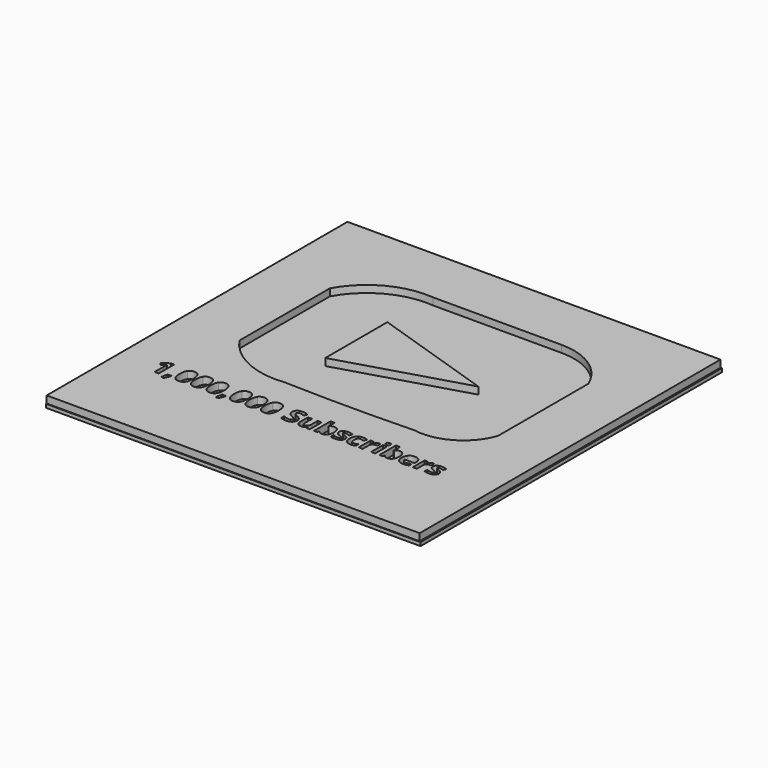
from build123d import *

# Parameters (mm, degrees)
F0_W         = 104.9293428659
F0_H         = 105.7772599161
F0_W_2       = 1.1398439379
F0_H_2       = 4.179029086
F1_DEPTH     = 3
F3_DEPTH     = 3
F4_W         = 105.3532995284
F4_H         = 105.9892401099
F5_DEPTH     = 1
F6_TEXT_SIZE = 5.2799160282
F7_DEPTH     = 1


# Not quite as in the source:
# - Text() gives the source's letters only with a copy of the font that has no kerning and outlines rounded to 1/6400 em; it was checked with that copy


with BuildPart() as f1:
    # F0 (on Top) → F1 (new body)
    with BuildSketch(Plane.XY):
        with Locations((-9.3270540237, 6.041387096)):
            Rectangle(F0_W, F0_H)
        with BuildLine():
            Line((-49.0903157705, -17.8528391492), (-49.0903157705, -23.3176313341))
            Line((-49.0903157705, -23.3176313341), (-50.2457084715, -23.3176313341))
            Line((-50.2457084715, -23.3176313341), (-50.2457084715, -20.1552521402))
            Line((-50.2457084715, -20.1552521402), (-50.2337478845, -19.6361626658))
            Line((-50.2337478845, -19.6361626658), (-50.2158070041, -19.0680347849))
            add(Edge.make_bspline(
                [(-50.2158070041, -19.0680347849), (-50.5028610912, -19.3550888721), (-50.6152906087, -19.4447932744)],
                knots=[0, 0, 0, 1, 1, 1], degree=2))
            Line((-50.6152906087, -19.4447932744), (-51.2432214245, -19.9495300444))
            Line((-51.2432214245, -19.9495300444), (-51.8005847771, -19.2546199416))
            Line((-51.8005847771, -19.2546199416), (-50.0399863756, -17.8528391492))
            Line((-50.0399863756, -17.8528391492), (-49.0903157705, -17.8528391492))
        make_face(mode=Mode.SUBTRACT)
        with BuildLine():
            Line((-46.2233630747, -22.4277636638), (-46.1683443747, -22.5138798899))
            add(Edge.make_bspline(
                [(-46.1683443747, -22.5138798899), (-46.3621058835, -23.2685929275), (-46.8261766578, -24.3043797588)],
                knots=[0, 0, 0, 1, 1, 1], degree=2))
            Line((-46.8261766578, -24.3043797588), (-47.6478689824, -24.3043797588))
            add(Edge.make_bspline(
                [(-47.6478689824, -24.3043797588), (-47.405069067, -23.3104549819), (-47.2699144343, -22.4277636638)],
                knots=[0, 0, 0, 1, 1, 1], degree=2))
            Line((-47.2699144343, -22.4277636638), (-46.2233630747, -22.4277636638))
        make_face(mode=Mode.SUBTRACT)
        with BuildLine():
            add(Edge.make_bspline(
                [(-42.0509123115, -18.484358141), (-41.5671065687, -19.201993359), (-41.5671065687, -20.585833271)],
                knots=[0, 0, 0, 1, 1, 1], degree=2))
            add(Edge.make_bspline(
                [(-41.5671065687, -20.585833271), (-41.5671065687, -22.0163194721), (-42.0359615778, -22.704651252)],
                knots=[0, 0, 0, 1, 1, 1], degree=2))
            add(Edge.make_bspline(
                [(-42.0359615778, -22.704651252), (-42.5048165869, -23.392983032), (-43.4808004833, -23.392983032)],
                knots=[0, 0, 0, 1, 1, 1], degree=2))
            add(Edge.make_bspline(
                [(-43.4808004833, -23.392983032), (-44.4268829124, -23.392983032), (-44.9071004791, -22.6825241662)],
                knots=[0, 0, 0, 1, 1, 1], degree=2))
            add(Edge.make_bspline(
                [(-44.9071004791, -22.6825241662), (-45.3873180458, -21.9720653004), (-45.3873180458, -20.585833271)],
                knots=[0, 0, 0, 1, 1, 1], degree=2))
            add(Edge.make_bspline(
                [(-45.3873180458, -20.585833271), (-45.3873180458, -19.1386022481), (-44.9196590954, -18.4526625855)],
                knots=[0, 0, 0, 1, 1, 1], degree=2))
            add(Edge.make_bspline(
                [(-44.9196590954, -18.4526625855), (-44.452000145, -17.766722923), (-43.4808004833, -17.766722923)],
                knots=[0, 0, 0, 1, 1, 1], degree=2))
            add(Edge.make_bspline(
                [(-43.4808004833, -17.766722923), (-42.5347180543, -17.766722923), (-42.0509123115, -18.484358141)],
                knots=[0, 0, 0, 1, 1, 1], degree=2))
        make_face(mode=Mode.SUBTRACT)
        with BuildLine():
            add(Edge.make_bspline(
                [(-37.6817098927, -18.484358141), (-37.19790415, -19.201993359), (-37.19790415, -20.585833271)],
                knots=[0, 0, 0, 1, 1, 1], degree=2))
            add(Edge.make_bspline(
                [(-37.19790415, -20.585833271), (-37.19790415, -22.0163194721), (-37.666759159, -22.704651252)],
                knots=[0, 0, 0, 1, 1, 1], degree=2))
            add(Edge.make_bspline(
                [(-37.666759159, -22.704651252), (-38.1356141681, -23.392983032), (-39.1115980646, -23.392983032)],
                knots=[0, 0, 0, 1, 1, 1], degree=2))
            add(Edge.make_bspline(
                [(-39.1115980646, -23.392983032), (-40.0576804936, -23.392983032), (-40.5378980603, -22.6825241662)],
                knots=[0, 0, 0, 1, 1, 1], degree=2))
            add(Edge.make_bspline(
                [(-40.5378980603, -22.6825241662), (-41.018115627, -21.9720653004), (-41.018115627, -20.585833271)],
                knots=[0, 0, 0, 1, 1, 1], degree=2))
            add(Edge.make_bspline(
                [(-41.018115627, -20.585833271), (-41.018115627, -19.1386022481), (-40.5504566766, -18.4526625855)],
                knots=[0, 0, 0, 1, 1, 1], degree=2))
            add(Edge.make_bspline(
                [(-40.5504566766, -18.4526625855), (-40.0827977262, -17.766722923), (-39.1115980646, -17.766722923)],
                knots=[0, 0, 0, 1, 1, 1], degree=2))
            add(Edge.make_bspline(
                [(-39.1115980646, -17.766722923), (-38.1655156355, -17.766722923), (-37.6817098927, -18.484358141)],
                knots=[0, 0, 0, 1, 1, 1], degree=2))
        make_face(mode=Mode.SUBTRACT)
        with BuildLine():
            add(Edge.make_bspline(
                [(-33.312507474, -18.484358141), (-32.8287017312, -19.201993359), (-32.8287017312, -20.585833271)],
                knots=[0, 0, 0, 1, 1, 1], degree=2))
            add(Edge.make_bspline(
                [(-32.8287017312, -20.585833271), (-32.8287017312, -22.0163194721), (-33.2975567403, -22.704651252)],
                knots=[0, 0, 0, 1, 1, 1], degree=2))
            add(Edge.make_bspline(
                [(-33.2975567403, -22.704651252), (-33.7664117493, -23.392983032), (-34.7423956458, -23.392983032)],
                knots=[0, 0, 0, 1, 1, 1], degree=2))
            add(Edge.make_bspline(
                [(-34.7423956458, -23.392983032), (-35.6884780748, -23.392983032), (-36.1686956415, -22.6825241662)],
                knots=[0, 0, 0, 1, 1, 1], degree=2))
            add(Edge.make_bspline(
                [(-36.1686956415, -22.6825241662), (-36.6489132082, -21.9720653004), (-36.6489132082, -20.585833271)],
                knots=[0, 0, 0, 1, 1, 1], degree=2))
            add(Edge.make_bspline(
                [(-36.6489132082, -20.585833271), (-36.6489132082, -19.1386022481), (-36.1812542578, -18.4526625855)],
                knots=[0, 0, 0, 1, 1, 1], degree=2))
            add(Edge.make_bspline(
                [(-36.1812542578, -18.4526625855), (-35.7135953074, -17.766722923), (-34.7423956458, -17.766722923)],
                knots=[0, 0, 0, 1, 1, 1], degree=2))
            add(Edge.make_bspline(
                [(-34.7423956458, -17.766722923), (-33.7963132168, -17.766722923), (-33.312507474, -18.484358141)],
                knots=[0, 0, 0, 1, 1, 1], degree=2))
        make_face(mode=Mode.SUBTRACT)
        with BuildLine():
            Line((-30.8958708774, -22.4277636638), (-30.8408521774, -22.5138798899))
            add(Edge.make_bspline(
                [(-30.8408521774, -22.5138798899), (-31.0346136862, -23.2685929275), (-31.4986844605, -24.3043797588)],
                knots=[0, 0, 0, 1, 1, 1], degree=2))
            Line((-31.4986844605, -24.3043797588), (-32.3203767851, -24.3043797588))
            add(Edge.make_bspline(
                [(-32.3203767851, -24.3043797588), (-32.0775768697, -23.3104549819), (-31.942422237, -22.4277636638)],
                knots=[0, 0, 0, 1, 1, 1], degree=2))
            Line((-31.942422237, -22.4277636638), (-30.8958708774, -22.4277636638))
        make_face(mode=Mode.SUBTRACT)
        with BuildLine():
            add(Edge.make_bspline(
                [(-26.7234201142, -18.484358141), (-26.2396143715, -19.201993359), (-26.2396143715, -20.585833271)],
                knots=[0, 0, 0, 1, 1, 1], degree=2))
            add(Edge.make_bspline(
                [(-26.2396143715, -20.585833271), (-26.2396143715, -22.0163194721), (-26.7084693805, -22.704651252)],
                knots=[0, 0, 0, 1, 1, 1], degree=2))
            add(Edge.make_bspline(
                [(-26.7084693805, -22.704651252), (-27.1773243896, -23.392983032), (-28.1533082861, -23.392983032)],
                knots=[0, 0, 0, 1, 1, 1], degree=2))
            add(Edge.make_bspline(
                [(-28.1533082861, -23.392983032), (-29.0993907151, -23.392983032), (-29.5796082818, -22.6825241662)],
                knots=[0, 0, 0, 1, 1, 1], degree=2))
            add(Edge.make_bspline(
                [(-29.5796082818, -22.6825241662), (-30.0598258485, -21.9720653004), (-30.0598258485, -20.585833271)],
                knots=[0, 0, 0, 1, 1, 1], degree=2))
            add(Edge.make_bspline(
                [(-30.0598258485, -20.585833271), (-30.0598258485, -19.1386022481), (-29.5921668981, -18.4526625855)],
                knots=[0, 0, 0, 1, 1, 1], degree=2))
            add(Edge.make_bspline(
                [(-29.5921668981, -18.4526625855), (-29.1245079477, -17.766722923), (-28.1533082861, -17.766722923)],
                knots=[0, 0, 0, 1, 1, 1], degree=2))
            add(Edge.make_bspline(
                [(-28.1533082861, -17.766722923), (-27.207225857, -17.766722923), (-26.7234201142, -18.484358141)],
                knots=[0, 0, 0, 1, 1, 1], degree=2))
        make_face(mode=Mode.SUBTRACT)
        with BuildLine():
            add(Edge.make_bspline(
                [(-22.3542176955, -18.484358141), (-21.8704119527, -19.201993359), (-21.8704119527, -20.585833271)],
                knots=[0, 0, 0, 1, 1, 1], degree=2))
            add(Edge.make_bspline(
                [(-21.8704119527, -20.585833271), (-21.8704119527, -22.0163194721), (-22.3392669618, -22.704651252)],
                knots=[0, 0, 0, 1, 1, 1], degree=2))
            add(Edge.make_bspline(
                [(-22.3392669618, -22.704651252), (-22.8081219708, -23.392983032), (-23.7841058673, -23.392983032)],
                knots=[0, 0, 0, 1, 1, 1], degree=2))
            add(Edge.make_bspline(
                [(-23.7841058673, -23.392983032), (-24.7301882963, -23.392983032), (-25.210405863, -22.6825241662)],
                knots=[0, 0, 0, 1, 1, 1], degree=2))
            add(Edge.make_bspline(
                [(-25.210405863, -22.6825241662), (-25.6906234297, -21.9720653004), (-25.6906234297, -20.585833271)],
                knots=[0, 0, 0, 1, 1, 1], degree=2))
            add(Edge.make_bspline(
                [(-25.6906234297, -20.585833271), (-25.6906234297, -19.1386022481), (-25.2229644793, -18.4526625855)],
                knots=[0, 0, 0, 1, 1, 1], degree=2))
            add(Edge.make_bspline(
                [(-25.2229644793, -18.4526625855), (-24.7553055289, -17.766722923), (-23.7841058673, -17.766722923)],
                knots=[0, 0, 0, 1, 1, 1], degree=2))
            add(Edge.make_bspline(
                [(-23.7841058673, -17.766722923), (-22.8380234383, -17.766722923), (-22.3542176955, -18.484358141)],
                knots=[0, 0, 0, 1, 1, 1], degree=2))
        make_face(mode=Mode.SUBTRACT)
        with BuildLine():
            add(Edge.make_bspline(
                [(-17.9850152767, -18.484358141), (-17.5012095339, -19.201993359), (-17.5012095339, -20.585833271)],
                knots=[0, 0, 0, 1, 1, 1], degree=2))
            add(Edge.make_bspline(
                [(-17.5012095339, -20.585833271), (-17.5012095339, -22.0163194721), (-17.970064543, -22.704651252)],
                knots=[0, 0, 0, 1, 1, 1], degree=2))
            add(Edge.make_bspline(
                [(-17.970064543, -22.704651252), (-18.4389195521, -23.392983032), (-19.4149034485, -23.392983032)],
                knots=[0, 0, 0, 1, 1, 1], degree=2))
            add(Edge.make_bspline(
                [(-19.4149034485, -23.392983032), (-20.3609858775, -23.392983032), (-20.8412034442, -22.6825241662)],
                knots=[0, 0, 0, 1, 1, 1], degree=2))
            add(Edge.make_bspline(
                [(-20.8412034442, -22.6825241662), (-21.3214210109, -21.9720653004), (-21.3214210109, -20.585833271)],
                knots=[0, 0, 0, 1, 1, 1], degree=2))
            add(Edge.make_bspline(
                [(-21.3214210109, -20.585833271), (-21.3214210109, -19.1386022481), (-20.8537620605, -18.4526625855)],
                knots=[0, 0, 0, 1, 1, 1], degree=2))
            add(Edge.make_bspline(
                [(-20.8537620605, -18.4526625855), (-20.3861031102, -17.766722923), (-19.4149034485, -17.766722923)],
                knots=[0, 0, 0, 1, 1, 1], degree=2))
            add(Edge.make_bspline(
                [(-19.4149034485, -17.766722923), (-18.4688210195, -17.766722923), (-17.9850152767, -18.484358141)],
                knots=[0, 0, 0, 1, 1, 1], degree=2))
        make_face(mode=Mode.SUBTRACT)
        with BuildLine():
            add(Edge.make_bspline(
                [(-11.6100224237, -20.8974065614), (-11.3259584832, -21.2651946107), (-11.3259584832, -21.799832848)],
                knots=[0, 0, 0, 1, 1, 1], degree=2))
            add(Edge.make_bspline(
                [(-11.3259584832, -21.799832848), (-11.3259584832, -22.5401931813), (-11.8588026326, -22.9665881066)],
                knots=[0, 0, 0, 1, 1, 1], degree=2))
            add(Edge.make_bspline(
                [(-11.8588026326, -22.9665881066), (-12.3916467819, -23.392983032), (-13.3401213283, -23.392983032)],
                knots=[0, 0, 0, 1, 1, 1], degree=2))
            add(Edge.make_bspline(
                [(-13.3401213283, -23.392983032), (-14.2156362943, -23.392983032), (-14.8878212818, -23.0628708317)],
                knots=[0, 0, 0, 1, 1, 1], degree=2))
            Line((-14.8878212818, -23.0628708317), (-14.8878212818, -21.9864180047))
            add(Edge.make_bspline(
                [(-14.8878212818, -21.9864180047), (-14.3352421639, -22.2340021549), (-13.9519053517, -22.3344710854)],
                knots=[0, 0, 0, 1, 1, 1], degree=2))
            add(Edge.make_bspline(
                [(-13.9519053517, -22.3344710854), (-13.5685685394, -22.434940016), (-13.2504169261, -22.434940016)],
                knots=[0, 0, 0, 1, 1, 1], degree=2))
            add(Edge.make_bspline(
                [(-13.2504169261, -22.434940016), (-12.8700702606, -22.434940016), (-12.6661422528, -22.2896188843)],
                knots=[0, 0, 0, 1, 1, 1], degree=2))
            add(Edge.make_bspline(
                [(-12.6661422528, -22.2896188843), (-12.462214245, -22.1442977527), (-12.462214245, -21.8560476068)],
                knots=[0, 0, 0, 1, 1, 1], degree=2))
            add(Edge.make_bspline(
                [(-12.462214245, -21.8560476068), (-12.462214245, -21.6957757414), (-12.5519186473, -21.5701895783)],
                knots=[0, 0, 0, 1, 1, 1], degree=2))
            add(Edge.make_bspline(
                [(-12.5519186473, -21.5701895783), (-12.6416230495, -21.4446034151), (-12.8156495899, -21.3291837509)],
                knots=[0, 0, 0, 1, 1, 1], degree=2))
            add(Edge.make_bspline(
                [(-12.8156495899, -21.3291837509), (-12.9896761302, -21.2137640867), (-13.5243143676, -20.9590035843)],
                knots=[0, 0, 0, 1, 1, 1], degree=2))
            add(Edge.make_bspline(
                [(-13.5243143676, -20.9590035843), (-14.0242669028, -20.7233800211), (-14.2748411997, -20.506893397)],
                knots=[0, 0, 0, 1, 1, 1], degree=2))
            add(Edge.make_bspline(
                [(-14.2748411997, -20.506893397), (-14.5254154967, -20.2904067729), (-14.6749228338, -20.002156627)],
                knots=[0, 0, 0, 1, 1, 1], degree=2))
            add(Edge.make_bspline(
                [(-14.6749228338, -20.002156627), (-14.8244301708, -19.7139064811), (-14.8244301708, -19.3299716395)],
                knots=[0, 0, 0, 1, 1, 1], degree=2))
            add(Edge.make_bspline(
                [(-14.8244301708, -19.3299716395), (-14.8244301708, -18.6039640107), (-14.3328500465, -18.1895296723)],
                knots=[0, 0, 0, 1, 1, 1], degree=2))
            add(Edge.make_bspline(
                [(-14.3328500465, -18.1895296723), (-13.8412699222, -17.7750953339), (-12.9741273672, -17.7750953339)],
                knots=[0, 0, 0, 1, 1, 1], degree=2))
            add(Edge.make_bspline(
                [(-12.9741273672, -17.7750953339), (-12.5483304712, -17.7750953339), (-12.1614054828, -17.8755642644)],
                knots=[0, 0, 0, 1, 1, 1], degree=2))
            add(Edge.make_bspline(
                [(-12.1614054828, -17.8755642644), (-11.7744804944, -17.9760331949), (-11.3522717745, -18.1590301755)],
                knots=[0, 0, 0, 1, 1, 1], degree=2))
            Line((-11.3522717745, -18.1590301755), (-11.7254420879, -19.0608584328))
            add(Edge.make_bspline(
                [(-11.7254420879, -19.0608584328), (-12.1631995709, -18.8814496283), (-12.4490575993, -18.8102841358)],
                knots=[0, 0, 0, 1, 1, 1], degree=2))
            add(Edge.make_bspline(
                [(-12.4490575993, -18.8102841358), (-12.7349156278, -18.7391186434), (-13.0112051868, -18.7391186434)],
                knots=[0, 0, 0, 1, 1, 1], degree=2))
            add(Edge.make_bspline(
                [(-13.0112051868, -18.7391186434), (-13.3401213283, -18.7391186434), (-13.5159419567, -18.8922141565)],
                knots=[0, 0, 0, 1, 1, 1], degree=2))
            add(Edge.make_bspline(
                [(-13.5159419567, -18.8922141565), (-13.6917625851, -19.0453096697), (-13.6917625851, -19.2916977612)],
                knots=[0, 0, 0, 1, 1, 1], degree=2))
            add(Edge.make_bspline(
                [(-13.6917625851, -19.2916977612), (-13.6917625851, -19.4447932744), (-13.6205970927, -19.5590168799)],
                knots=[0, 0, 0, 1, 1, 1], degree=2))
            add(Edge.make_bspline(
                [(-13.6205970927, -19.5590168799), (-13.5494316002, -19.6732404854), (-13.394541999, -19.7796897094)],
                knots=[0, 0, 0, 1, 1, 1], degree=2))
            add(Edge.make_bspline(
                [(-13.394541999, -19.7796897094), (-13.2396523978, -19.8861389334), (-12.6607599886, -20.1624284924)],
                knots=[0, 0, 0, 1, 1, 1], degree=2))
            add(Edge.make_bspline(
                [(-12.6607599886, -20.1624284924), (-11.8940863641, -20.5296185122), (-11.6100224237, -20.8974065614)],
                knots=[0, 0, 0, 1, 1, 1], degree=2))
        make_face(mode=Mode.SUBTRACT)
        with BuildLine():
            Line((-6.5907621033, -23.3176313341), (-7.4650810105, -23.3176313341))
            Line((-7.4650810105, -23.3176313341), (-7.6181765237, -22.7829930967))
            Line((-7.6181765237, -22.7829930967), (-7.6779794585, -22.7829930967))
            add(Edge.make_bspline(
                [(-7.6779794585, -22.7829930967), (-7.8609764391, -23.0748314187), (-8.1976669622, -23.2339072253)],
                knots=[0, 0, 0, 1, 1, 1], degree=2))
            add(Edge.make_bspline(
                [(-8.1976669622, -23.2339072253), (-8.5343574853, -23.392983032), (-8.9637425574, -23.392983032)],
                knots=[0, 0, 0, 1, 1, 1], degree=2))
            add(Edge.make_bspline(
                [(-8.9637425574, -23.392983032), (-9.7005147145, -23.392983032), (-10.0742830572, -22.9982836621)],
                knots=[0, 0, 0, 1, 1, 1], degree=2))
            add(Edge.make_bspline(
                [(-10.0742830572, -22.9982836621), (-10.4480513999, -22.6035842922), (-10.4480513999, -21.863223959)],
                knots=[0, 0, 0, 1, 1, 1], degree=2))
            Line((-10.4480513999, -21.863223959), (-10.4480513999, -19.1386022481))
            Line((-10.4480513999, -19.1386022481), (-9.308207462, -19.1386022481))
            Line((-9.308207462, -19.1386022481), (-9.308207462, -21.5797580479))
            add(Edge.make_bspline(
                [(-9.308207462, -21.5797580479), (-9.308207462, -22.0318682352), (-9.1473375673, -22.2579233289)],
                knots=[0, 0, 0, 1, 1, 1], degree=2))
            add(Edge.make_bspline(
                [(-9.1473375673, -22.2579233289), (-8.9864676726, -22.4839784225), (-8.6348264158, -22.4839784225)],
                knots=[0, 0, 0, 1, 1, 1], degree=2))
            add(Edge.make_bspline(
                [(-8.6348264158, -22.4839784225), (-8.1564029371, -22.4839784225), (-7.9435044891, -22.1646307505)],
                knots=[0, 0, 0, 1, 1, 1], degree=2))
            add(Edge.make_bspline(
                [(-7.9435044891, -22.1646307505), (-7.7306060412, -21.8452830785), (-7.7306060412, -21.1049227453)],
                knots=[0, 0, 0, 1, 1, 1], degree=2))
            Line((-7.7306060412, -21.1049227453), (-7.7306060412, -19.1386022481))
            Line((-7.7306060412, -19.1386022481), (-6.5907621033, -19.1386022481))
            Line((-6.5907621033, -19.1386022481), (-6.5907621033, -23.3176313341))
        make_face(mode=Mode.SUBTRACT)
        with BuildLine():
            add(Edge.make_bspline(
                [(-4.2548594688, -19.6804168376), (-3.8541798054, -19.0608584328), (-3.0695653004, -19.0608584328)],
                knots=[0, 0, 0, 1, 1, 1], degree=2))
            add(Edge.make_bspline(
                [(-3.0695653004, -19.0608584328), (-2.3292049672, -19.0608584328), (-1.9105844234, -19.6379567539)],
                knots=[0, 0, 0, 1, 1, 1], degree=2))
            add(Edge.make_bspline(
                [(-1.9105844234, -19.6379567539), (-1.4919638795, -20.215055075), (-1.4919638795, -21.2209404389)],
                knots=[0, 0, 0, 1, 1, 1], degree=2))
            add(Edge.make_bspline(
                [(-1.4919638795, -21.2209404389), (-1.4919638795, -22.2555312115), (-1.923741069, -22.8242571217)],
                knots=[0, 0, 0, 1, 1, 1], degree=2))
            add(Edge.make_bspline(
                [(-1.923741069, -22.8242571217), (-2.3555182585, -23.392983032), (-3.0994667678, -23.392983032)],
                knots=[0, 0, 0, 1, 1, 1], degree=2))
            add(Edge.make_bspline(
                [(-3.0994667678, -23.392983032), (-3.8362389249, -23.392983032), (-4.2548594688, -22.8583447946)],
                knots=[0, 0, 0, 1, 1, 1], degree=2))
            Line((-4.2548594688, -22.8583447946), (-4.332603284, -22.8583447946))
            Line((-4.332603284, -22.8583447946), (-4.5239726755, -23.3176313341))
            Line((-4.5239726755, -23.3176313341), (-5.3947034066, -23.3176313341))
            Line((-5.3947034066, -23.3176313341), (-5.3947034066, -17.5011978924))
            Line((-5.3947034066, -17.5011978924), (-4.2548594688, -17.5011978924))
            Line((-4.2548594688, -17.5011978924), (-4.2548594688, -18.8551363369))
            add(Edge.make_bspline(
                [(-4.2548594688, -18.8551363369), (-4.2548594688, -19.1122889567), (-4.2991136405, -19.6804168376)],
                knots=[0, 0, 0, 1, 1, 1], degree=2))
            Line((-4.2991136405, -19.6804168376), (-4.2548594688, -19.6804168376))
        make_face(mode=Mode.SUBTRACT)
        with BuildLine():
            add(Edge.make_bspline(
                [(2.2564840757, -21.5420821989), (2.3653254171, -21.7663432045), (2.3653254171, -22.076122407)],
                knots=[0, 0, 0, 1, 1, 1], degree=2))
            add(Edge.make_bspline(
                [(2.3653254171, -22.076122407), (2.3653254171, -22.7196019858), (1.9185974939, -23.0562925089)],
                knots=[0, 0, 0, 1, 1, 1], degree=2))
            add(Edge.make_bspline(
                [(1.9185974939, -23.0562925089), (1.4718695707, -23.392983032), (0.5820019004, -23.392983032)],
                knots=[0, 0, 0, 1, 1, 1], degree=2))
            add(Edge.make_bspline(
                [(0.5820019004, -23.392983032), (0.126303537, -23.392983032), (-0.1954362524, -23.3307879797)],
                knots=[0, 0, 0, 1, 1, 1], degree=2))
            add(Edge.make_bspline(
                [(-0.1954362524, -23.3307879797), (-0.5171760418, -23.2685929275), (-0.7970537768, -23.1489870578)],
                knots=[0, 0, 0, 1, 1, 1], degree=2))
            Line((-0.7970537768, -23.1489870578), (-0.7970537768, -22.2076888636))
            add(Edge.make_bspline(
                [(-0.7970537768, -22.2076888636), (-0.4800982222, -22.3571962007), (-0.0818106762, -22.4582631605)],
                knots=[0, 0, 0, 1, 1, 1], degree=2))
            add(Edge.make_bspline(
                [(-0.0818106762, -22.4582631605), (0.3164768698, -22.5593301204), (0.61907972, -22.5593301204)],
                knots=[0, 0, 0, 1, 1, 1], degree=2))
            add(Edge.make_bspline(
                [(0.61907972, -22.5593301204), (1.2398341836, -22.5593301204), (1.2398341836, -22.2005125114)],
                knots=[0, 0, 0, 1, 1, 1], degree=2))
            add(Edge.make_bspline(
                [(1.2398341836, -22.2005125114), (1.2398341836, -22.0653578787), (1.1573061335, -21.9810357406)],
                knots=[0, 0, 0, 1, 1, 1], degree=2))
            add(Edge.make_bspline(
                [(1.1573061335, -21.9810357406), (1.0747780834, -21.8967136025), (0.873242193, -21.7902643785)],
                knots=[0, 0, 0, 1, 1, 1], degree=2))
            add(Edge.make_bspline(
                [(0.873242193, -21.7902643785), (0.6717063027, -21.6838151545), (0.3356138089, -21.5426802283)],
                knots=[0, 0, 0, 1, 1, 1], degree=2))
            add(Edge.make_bspline(
                [(0.3356138089, -21.5426802283), (-0.1463978458, -21.3405463085), (-0.3730509688, -21.1683138562)],
                knots=[0, 0, 0, 1, 1, 1], degree=2))
            add(Edge.make_bspline(
                [(-0.3730509688, -21.1683138562), (-0.5997040919, -20.9960814039), (-0.7019671104, -20.7736144863)],
                knots=[0, 0, 0, 1, 1, 1], degree=2))
            add(Edge.make_bspline(
                [(-0.7019671104, -20.7736144863), (-0.804230129, -20.5511475688), (-0.804230129, -20.227015662)],
                knots=[0, 0, 0, 1, 1, 1], degree=2))
            add(Edge.make_bspline(
                [(-0.804230129, -20.227015662), (-0.804230129, -19.6696523094), (-0.3730509688, -19.3652553711)],
                knots=[0, 0, 0, 1, 1, 1], degree=2))
            add(Edge.make_bspline(
                [(-0.3730509688, -19.3652553711), (0.0581281913, -19.0608584328), (0.8511151072, -19.0608584328)],
                knots=[0, 0, 0, 1, 1, 1], degree=2))
            add(Edge.make_bspline(
                [(0.8511151072, -19.0608584328), (1.6058281447, -19.0608584328), (2.3198751866, -19.3897745743)],
                knots=[0, 0, 0, 1, 1, 1], degree=2))
            Line((2.3198751866, -19.3897745743), (1.9766063407, -20.2114668989))
            add(Edge.make_bspline(
                [(1.9766063407, -20.2114668989), (1.6620429035, -20.0775083249), (1.3893415206, -19.9913920987)],
                knots=[0, 0, 0, 1, 1, 1], degree=2))
            add(Edge.make_bspline(
                [(1.3893415206, -19.9913920987), (1.1166401378, -19.9052758726), (0.831978168, -19.9052758726)],
                knots=[0, 0, 0, 1, 1, 1], degree=2))
            add(Edge.make_bspline(
                [(0.831978168, -19.9052758726), (0.327241398, -19.9052758726), (0.327241398, -20.1779772554)],
                knots=[0, 0, 0, 1, 1, 1], degree=2))
            add(Edge.make_bspline(
                [(0.327241398, -20.1779772554), (0.327241398, -20.3310727686), (0.4899053808, -20.4435022861)],
                knots=[0, 0, 0, 1, 1, 1], degree=2))
            add(Edge.make_bspline(
                [(0.4899053808, -20.4435022861), (0.6525693635, -20.5559318036), (1.202756364, -20.7760066037)],
                knots=[0, 0, 0, 1, 1, 1], degree=2))
            add(Edge.make_bspline(
                [(1.202756364, -20.7760066037), (1.6919443709, -20.9745523474), (1.9197935526, -21.1461867703)],
                knots=[0, 0, 0, 1, 1, 1], degree=2))
            add(Edge.make_bspline(
                [(1.9197935526, -21.1461867703), (2.1476427343, -21.3178211933), (2.2564840757, -21.5420821989)],
                knots=[0, 0, 0, 1, 1, 1], degree=2))
        make_face(mode=Mode.SUBTRACT)
        with BuildLine():
            add(Edge.make_bspline(
                [(5.6628592437, -23.3254057156), (5.3805893913, -23.392983032), (4.9512043192, -23.392983032)],
                knots=[0, 0, 0, 1, 1, 1], degree=2))
            add(Edge.make_bspline(
                [(4.9512043192, -23.392983032), (3.000432585, -23.392983032), (3.000432585, -21.2508419063)],
                knots=[0, 0, 0, 1, 1, 1], degree=2))
            add(Edge.make_bspline(
                [(3.000432585, -21.2508419063), (3.000432585, -20.1851536076), (3.5308846169, -19.6230060202)],
                knots=[0, 0, 0, 1, 1, 1], degree=2))
            add(Edge.make_bspline(
                [(3.5308846169, -19.6230060202), (4.0613366489, -19.0608584328), (5.0516732497, -19.0608584328)],
                knots=[0, 0, 0, 1, 1, 1], degree=2))
            add(Edge.make_bspline(
                [(5.0516732497, -19.0608584328), (5.7764848199, -19.0608584328), (6.3529851116, -19.3443243439)],
                knots=[0, 0, 0, 1, 1, 1], degree=2))
            Line((6.3529851116, -19.3443243439), (6.0156965592, -20.227015662))
            add(Edge.make_bspline(
                [(6.0156965592, -20.227015662), (5.7465833524, -20.1181743206), (5.5151459947, -20.0488029162)],
                knots=[0, 0, 0, 1, 1, 1], degree=2))
            add(Edge.make_bspline(
                [(5.5151459947, -20.0488029162), (5.2837086369, -19.9794315118), (5.0516732497, -19.9794315118)],
                knots=[0, 0, 0, 1, 1, 1], degree=2))
            add(Edge.make_bspline(
                [(5.0516732497, -19.9794315118), (4.1618055794, -19.9794315118), (4.1618055794, -21.2436655541)],
                knots=[0, 0, 0, 1, 1, 1], degree=2))
            add(Edge.make_bspline(
                [(4.1618055794, -21.2436655541), (4.1618055794, -22.4696257182), (5.0516732497, -22.4696257182)],
                knots=[0, 0, 0, 1, 1, 1], degree=2))
            add(Edge.make_bspline(
                [(5.0516732497, -22.4696257182), (5.3805893913, -22.4696257182), (5.6610651556, -22.381715404)],
                knots=[0, 0, 0, 1, 1, 1], degree=2))
            add(Edge.make_bspline(
                [(5.6610651556, -22.381715404), (5.94154092, -22.2938050898), (6.221418655, -22.1060238744)],
                knots=[0, 0, 0, 1, 1, 1], degree=2))
            Line((6.221418655, -22.1060238744), (6.221418655, -23.0820077708))
            add(Edge.make_bspline(
                [(6.221418655, -23.0820077708), (5.9451290961, -23.2578283992), (5.6628592437, -23.3254057156)],
                knots=[0, 0, 0, 1, 1, 1], degree=2))
        make_face(mode=Mode.SUBTRACT)
        with BuildLine():
            add(Edge.make_bspline(
                [(8.8031113517, -19.2755509688), (9.1338215813, -19.0608584328), (9.5225406577, -19.0608584328)],
                knots=[0, 0, 0, 1, 1, 1], degree=2))
            add(Edge.make_bspline(
                [(9.5225406577, -19.0608584328), (9.7545760448, -19.0608584328), (9.907671558, -19.0943480763)],
                knots=[0, 0, 0, 1, 1, 1], degree=2))
            Line((9.907671558, -19.0943480763), (9.8215553319, -20.1624284924))
            add(Edge.make_bspline(
                [(9.8215553319, -20.1624284924), (9.682812523, -20.1253506728), (9.4854628381, -20.1253506728)],
                knots=[0, 0, 0, 1, 1, 1], degree=2))
            add(Edge.make_bspline(
                [(9.4854628381, -20.1253506728), (8.9400600724, -20.1253506728), (8.6350651048, -20.4058264371)],
                knots=[0, 0, 0, 1, 1, 1], degree=2))
            add(Edge.make_bspline(
                [(8.6350651048, -20.4058264371), (8.3300701372, -20.6863022015), (8.3300701372, -21.1910389715)],
                knots=[0, 0, 0, 1, 1, 1], degree=2))
            Line((8.3300701372, -21.1910389715), (8.3300701372, -23.3176313341))
            Line((8.3300701372, -23.3176313341), (7.1902261993, -23.3176313341))
            Line((7.1902261993, -23.3176313341), (7.1902261993, -19.1386022481))
            Line((7.1902261993, -19.1386022481), (8.0537805782, -19.1386022481))
            Line((8.0537805782, -19.1386022481), (8.2224248545, -19.8418847617))
            Line((8.2224248545, -19.8418847617), (8.2774435545, -19.8418847617))
            add(Edge.make_bspline(
                [(8.2774435545, -19.8418847617), (8.4724011221, -19.4902435049), (8.8031113517, -19.2755509688)],
                knots=[0, 0, 0, 1, 1, 1], degree=2))
        make_face(mode=Mode.SUBTRACT)
        with Locations((11.2358947406, -21.2281167911)):
            Rectangle(F0_W_2, F0_H_2, mode=Mode.SUBTRACT)
        with BuildLine():
            add(Edge.make_bspline(
                [(14.1417193441, -19.6804168376), (14.5423990074, -19.0608584328), (15.3270135124, -19.0608584328)],
                knots=[0, 0, 0, 1, 1, 1], degree=2))
            add(Edge.make_bspline(
                [(15.3270135124, -19.0608584328), (16.0673738456, -19.0608584328), (16.4859943895, -19.6379567539)],
                knots=[0, 0, 0, 1, 1, 1], degree=2))
            add(Edge.make_bspline(
                [(16.4859943895, -19.6379567539), (16.9046149333, -20.215055075), (16.9046149333, -21.2209404389)],
                knots=[0, 0, 0, 1, 1, 1], degree=2))
            add(Edge.make_bspline(
                [(16.9046149333, -21.2209404389), (16.9046149333, -22.2555312115), (16.4728377438, -22.8242571217)],
                knots=[0, 0, 0, 1, 1, 1], degree=2))
            add(Edge.make_bspline(
                [(16.4728377438, -22.8242571217), (16.0410605543, -23.392983032), (15.297112045, -23.392983032)],
                knots=[0, 0, 0, 1, 1, 1], degree=2))
            add(Edge.make_bspline(
                [(15.297112045, -23.392983032), (14.5603398879, -23.392983032), (14.1417193441, -22.8583447946)],
                knots=[0, 0, 0, 1, 1, 1], degree=2))
            Line((14.1417193441, -22.8583447946), (14.0639755288, -22.8583447946))
            Line((14.0639755288, -22.8583447946), (13.8726061373, -23.3176313341))
            Line((13.8726061373, -23.3176313341), (13.0018754062, -23.3176313341))
            Line((13.0018754062, -23.3176313341), (13.0018754062, -17.5011978924))
            Line((13.0018754062, -17.5011978924), (14.1417193441, -17.5011978924))
            Line((14.1417193441, -17.5011978924), (14.1417193441, -18.8551363369))
            add(Edge.make_bspline(
                [(14.1417193441, -18.8551363369), (14.1417193441, -19.1122889567), (14.0974651723, -19.6804168376)],
                knots=[0, 0, 0, 1, 1, 1], degree=2))
            Line((14.0974651723, -19.6804168376), (14.1417193441, -19.6804168376))
        make_face(mode=Mode.SUBTRACT)
        with BuildLine():
            add(Edge.make_bspline(
                [(20.5669466624, -23.3200234515), (20.2272659925, -23.392983032), (19.7368819269, -23.392983032)],
                knots=[0, 0, 0, 1, 1, 1], degree=2))
            add(Edge.make_bspline(
                [(19.7368819269, -23.392983032), (18.7286044456, -23.392983032), (18.1604765647, -22.8356196793)],
                knots=[0, 0, 0, 1, 1, 1], degree=2))
            add(Edge.make_bspline(
                [(18.1604765647, -22.8356196793), (17.5923486838, -22.2782563267), (17.5923486838, -21.2580182585)],
                knots=[0, 0, 0, 1, 1, 1], degree=2))
            add(Edge.make_bspline(
                [(17.5923486838, -21.2580182585), (17.5923486838, -20.2078787228), (18.1174184517, -19.6343685778)],
                knots=[0, 0, 0, 1, 1, 1], degree=2))
            add(Edge.make_bspline(
                [(18.1174184517, -19.6343685778), (18.6424882195, -19.0608584328), (19.5694337094, -19.0608584328)],
                knots=[0, 0, 0, 1, 1, 1], degree=2))
            add(Edge.make_bspline(
                [(19.5694337094, -19.0608584328), (20.4545171449, -19.0608584328), (20.9478913572, -19.5649971734)],
                knots=[0, 0, 0, 1, 1, 1], degree=2))
            add(Edge.make_bspline(
                [(20.9478913572, -19.5649971734), (21.4412655696, -20.069135914), (21.4412655696, -20.9590035843)],
                knots=[0, 0, 0, 1, 1, 1], degree=2))
            Line((21.4412655696, -20.9590035843), (21.4412655696, -21.5127787609))
            Line((21.4412655696, -21.5127787609), (18.7465453261, -21.5127787609))
            add(Edge.make_bspline(
                [(18.7465453261, -21.5127787609), (18.7656822652, -21.9983785917), (19.034795472, -22.2710799745)],
                knots=[0, 0, 0, 1, 1, 1], degree=2))
            add(Edge.make_bspline(
                [(19.034795472, -22.2710799745), (19.3039086787, -22.5437813573), (19.7895085095, -22.5437813573)],
                knots=[0, 0, 0, 1, 1, 1], degree=2))
            add(Edge.make_bspline(
                [(19.7895085095, -22.5437813573), (20.1674630577, -22.5437813573), (20.5035555514, -22.4654395127)],
                knots=[0, 0, 0, 1, 1, 1], degree=2))
            add(Edge.make_bspline(
                [(20.5035555514, -22.4654395127), (20.8396480452, -22.3870976681), (21.2056420064, -22.2148652158)],
                knots=[0, 0, 0, 1, 1, 1], degree=2))
            Line((21.2056420064, -22.2148652158), (21.2056420064, -23.0975565339))
            add(Edge.make_bspline(
                [(21.2056420064, -23.0975565339), (20.9066273322, -23.247063871), (20.5669466624, -23.3200234515)],
                knots=[0, 0, 0, 1, 1, 1], degree=2))
        make_face(mode=Mode.SUBTRACT)
        with BuildLine():
            add(Edge.make_bspline(
                [(23.9810962119, -19.2755509688), (24.3118064415, -19.0608584328), (24.7005255179, -19.0608584328)],
                knots=[0, 0, 0, 1, 1, 1], degree=2))
            add(Edge.make_bspline(
                [(24.7005255179, -19.0608584328), (24.932560905, -19.0608584328), (25.0856564182, -19.0943480763)],
                knots=[0, 0, 0, 1, 1, 1], degree=2))
            Line((25.0856564182, -19.0943480763), (24.9995401921, -20.1624284924))
            add(Edge.make_bspline(
                [(24.9995401921, -20.1624284924), (24.8607973833, -20.1253506728), (24.6634476983, -20.1253506728)],
                knots=[0, 0, 0, 1, 1, 1], degree=2))
            add(Edge.make_bspline(
                [(24.6634476983, -20.1253506728), (24.1180449326, -20.1253506728), (23.813049965, -20.4058264371)],
                knots=[0, 0, 0, 1, 1, 1], degree=2))
            add(Edge.make_bspline(
                [(23.813049965, -20.4058264371), (23.5080549974, -20.6863022015), (23.5080549974, -21.1910389715)],
                knots=[0, 0, 0, 1, 1, 1], degree=2))
            Line((23.5080549974, -21.1910389715), (23.5080549974, -23.3176313341))
            Line((23.5080549974, -23.3176313341), (22.3682110595, -23.3176313341))
            Line((22.3682110595, -23.3176313341), (22.3682110595, -19.1386022481))
            Line((22.3682110595, -19.1386022481), (23.2317654384, -19.1386022481))
            Line((23.2317654384, -19.1386022481), (23.4004097147, -19.8418847617))
            Line((23.4004097147, -19.8418847617), (23.4554284147, -19.8418847617))
            add(Edge.make_bspline(
                [(23.4554284147, -19.8418847617), (23.6503859823, -19.4902435049), (23.9810962119, -19.2755509688)],
                knots=[0, 0, 0, 1, 1, 1], degree=2))
        make_face(mode=Mode.SUBTRACT)
        with BuildLine():
            add(Edge.make_bspline(
                [(28.6511073929, -21.5420821989), (28.7599487343, -21.7663432045), (28.7599487343, -22.076122407)],
                knots=[0, 0, 0, 1, 1, 1], degree=2))
            add(Edge.make_bspline(
                [(28.7599487343, -22.076122407), (28.7599487343, -22.7196019858), (28.3132208111, -23.0562925089)],
                knots=[0, 0, 0, 1, 1, 1], degree=2))
            add(Edge.make_bspline(
                [(28.3132208111, -23.0562925089), (27.8664928879, -23.392983032), (26.9766252176, -23.392983032)],
                knots=[0, 0, 0, 1, 1, 1], degree=2))
            add(Edge.make_bspline(
                [(26.9766252176, -23.392983032), (26.5209268542, -23.392983032), (26.1991870648, -23.3307879797)],
                knots=[0, 0, 0, 1, 1, 1], degree=2))
            add(Edge.make_bspline(
                [(26.1991870648, -23.3307879797), (25.8774472754, -23.2685929275), (25.5975695404, -23.1489870578)],
                knots=[0, 0, 0, 1, 1, 1], degree=2))
            Line((25.5975695404, -23.1489870578), (25.5975695404, -22.2076888636))
            add(Edge.make_bspline(
                [(25.5975695404, -22.2076888636), (25.914525095, -22.3571962007), (26.312812641, -22.4582631605)],
                knots=[0, 0, 0, 1, 1, 1], degree=2))
            add(Edge.make_bspline(
                [(26.312812641, -22.4582631605), (26.7111001869, -22.5593301204), (27.0137030372, -22.5593301204)],
                knots=[0, 0, 0, 1, 1, 1], degree=2))
            add(Edge.make_bspline(
                [(27.0137030372, -22.5593301204), (27.6344575007, -22.5593301204), (27.6344575007, -22.2005125114)],
                knots=[0, 0, 0, 1, 1, 1], degree=2))
            add(Edge.make_bspline(
                [(27.6344575007, -22.2005125114), (27.6344575007, -22.0653578787), (27.5519294507, -21.9810357406)],
                knots=[0, 0, 0, 1, 1, 1], degree=2))
            add(Edge.make_bspline(
                [(27.5519294507, -21.9810357406), (27.4694014006, -21.8967136025), (27.2678655102, -21.7902643785)],
                knots=[0, 0, 0, 1, 1, 1], degree=2))
            add(Edge.make_bspline(
                [(27.2678655102, -21.7902643785), (27.0663296198, -21.6838151545), (26.7302371261, -21.5426802283)],
                knots=[0, 0, 0, 1, 1, 1], degree=2))
            add(Edge.make_bspline(
                [(26.7302371261, -21.5426802283), (26.2482254713, -21.3405463085), (26.0215723483, -21.1683138562)],
                knots=[0, 0, 0, 1, 1, 1], degree=2))
            add(Edge.make_bspline(
                [(26.0215723483, -21.1683138562), (25.7949192253, -20.9960814039), (25.6926562068, -20.7736144863)],
                knots=[0, 0, 0, 1, 1, 1], degree=2))
            add(Edge.make_bspline(
                [(25.6926562068, -20.7736144863), (25.5903931882, -20.5511475688), (25.5903931882, -20.227015662)],
                knots=[0, 0, 0, 1, 1, 1], degree=2))
            add(Edge.make_bspline(
                [(25.5903931882, -20.227015662), (25.5903931882, -19.6696523094), (26.0215723483, -19.3652553711)],
                knots=[0, 0, 0, 1, 1, 1], degree=2))
            add(Edge.make_bspline(
                [(26.0215723483, -19.3652553711), (26.4527515085, -19.0608584328), (27.2457384243, -19.0608584328)],
                knots=[0, 0, 0, 1, 1, 1], degree=2))
            add(Edge.make_bspline(
                [(27.2457384243, -19.0608584328), (28.0004514619, -19.0608584328), (28.7144985038, -19.3897745743)],
                knots=[0, 0, 0, 1, 1, 1], degree=2))
            Line((28.7144985038, -19.3897745743), (28.3712296579, -20.2114668989))
            add(Edge.make_bspline(
                [(28.3712296579, -20.2114668989), (28.0566662206, -20.0775083249), (27.7839648378, -19.9913920987)],
                knots=[0, 0, 0, 1, 1, 1], degree=2))
            add(Edge.make_bspline(
                [(27.7839648378, -19.9913920987), (27.511263455, -19.9052758726), (27.2266014852, -19.9052758726)],
                knots=[0, 0, 0, 1, 1, 1], degree=2))
            add(Edge.make_bspline(
                [(27.2266014852, -19.9052758726), (26.7218647152, -19.9052758726), (26.7218647152, -20.1779772554)],
                knots=[0, 0, 0, 1, 1, 1], degree=2))
            add(Edge.make_bspline(
                [(26.7218647152, -20.1779772554), (26.7218647152, -20.3310727686), (26.8845286979, -20.4435022861)],
                knots=[0, 0, 0, 1, 1, 1], degree=2))
            add(Edge.make_bspline(
                [(26.8845286979, -20.4435022861), (27.0471926807, -20.5559318036), (27.5973796811, -20.7760066037)],
                knots=[0, 0, 0, 1, 1, 1], degree=2))
            add(Edge.make_bspline(
                [(27.5973796811, -20.7760066037), (28.0865676881, -20.9745523474), (28.3144168698, -21.1461867703)],
                knots=[0, 0, 0, 1, 1, 1], degree=2))
            add(Edge.make_bspline(
                [(28.3144168698, -21.1461867703), (28.5422660515, -21.3178211933), (28.6511073929, -21.5420821989)],
                knots=[0, 0, 0, 1, 1, 1], degree=2))
        make_face(mode=Mode.SUBTRACT)
        with BuildLine():
            add(Edge.make_bspline(
                [(11.2376888287, -18.6195127737), (10.6169343651, -18.6195127737), (10.6169343651, -18.058561245)],
                knots=[0, 0, 0, 1, 1, 1], degree=2))
            add(Edge.make_bspline(
                [(10.6169343651, -18.058561245), (10.6169343651, -17.5011978924), (11.2376888287, -17.5011978924)],
                knots=[0, 0, 0, 1, 1, 1], degree=2))
            add(Edge.make_bspline(
                [(11.2376888287, -17.5011978924), (11.8584432922, -17.5011978924), (11.8584432922, -18.058561245)],
                knots=[0, 0, 0, 1, 1, 1], degree=2))
            add(Edge.make_bspline(
                [(11.8584432922, -18.058561245), (11.8584432922, -18.3240862756), (11.703553691, -18.4717995247)],
                knots=[0, 0, 0, 1, 1, 1], degree=2))
            add(Edge.make_bspline(
                [(11.703553691, -18.4717995247), (11.5486640898, -18.6195127737), (11.2376888287, -18.6195127737)],
                knots=[0, 0, 0, 1, 1, 1], degree=2))
        make_face(mode=Mode.SUBTRACT)
        with BuildLine():
            ThreePointArc((-45.0454242527, 31.796772033), (-36.488463981, 40.2478812767), (-24.6954914182, 42.6076725125))
            Line((-24.6954914182, 42.6076725125), (11.5528292954, 42.6076725125))
            ThreePointArc((11.5528292954, 42.6076725125), (21.2535932932, 39.6544644958), (27.6631899178, 31.796772033))
            Line((27.6631899178, 31.796772033), (27.6631899178, 0))
            ThreePointArc((27.6631899178, 0), (21.3128083313, -7.6081781924), (11.5528292954, -9.3270530924))
            ThreePointArc((11.5528292954, -9.3270530924), (-6.5713310614, -9.6336374952), (-24.6954914182, -9.3270530924))
            ThreePointArc((-24.6954914182, -9.3270530924), (-36.1826145197, -7.5264136905), (-45.0454242527, 0))
            Line((-45.0454242527, 0), (-45.0454242527, 31.796772033))
        make_face(mode=Mode.SUBTRACT)
    extrude(amount=F1_DEPTH)


with BuildPart() as f3:
    # F2 (on Top) → F3 (new body)
    with BuildSketch(Plane.XY):
        Polygon((9.6450215206, 15.6864076853), (-25.1194480807, 27.1332450211), (-25.1194480807, 5.2994620055), align=None)
    extrude(amount=F3_DEPTH)


with BuildPart() as f5:
    # F4 (on Top) → F5 (new body)
    with BuildSketch(Plane.XY):
        with Locations((-9.1150756925, 5.9353969991)):
            Rectangle(F4_W, F4_H)
    extrude(amount=F5_DEPTH)


with BuildPart() as f7:
    # F6 (on Top) → F7 (new body)
    with BuildSketch(Plane.XY):
        with Locations((-59.2486262321, -33.5352867842)):
            Text('HAHAHA ITS JUST A PRANK BRO!!!', F6_TEXT_SIZE, font='Open Sans', text_align=(TextAlign.LEFT, TextAlign.BOTTOM))
    extrude(amount=F7_DEPTH)


solid = Compound([f1.part, f3.part, f5.part, f7.part])
